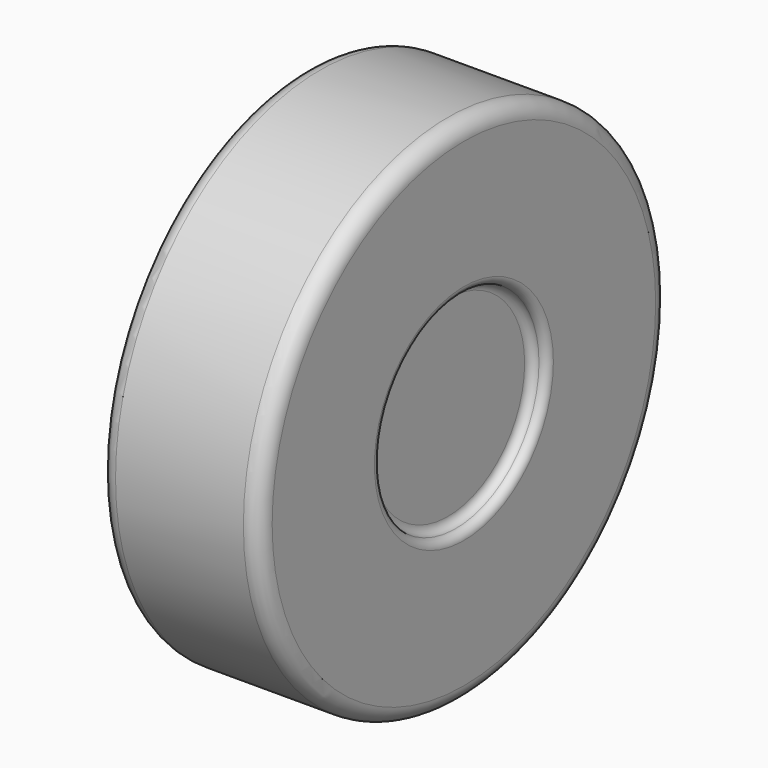
from build123d import *

# Parameters (mm, degrees)
F0_R     = 80
F1_DEPTH = 50
F2_R     = 32.5
F3_DEPTH = 5
F4_R     = 32.5
F5_DEPTH = 25
F6_R     = 5
F7_DEPTH = 10
F8_R     = 5
F9_R     = 2.49999


# Not quite as in the source:
# - a fillet or chamfer is up to 0.001 mm smaller than in the source, because OpenCascade refuses the exact size


with BuildPart() as f1:
    # F0 (on Right) → F1 (new body)
    with BuildSketch(Plane.YZ):
        Circle(F0_R)
    extrude(amount=F1_DEPTH)

    # F2 (on face) → F3 (cut)
    with BuildSketch(Plane.YZ.offset(50)):
        Circle(F2_R)
    extrude(amount=-F3_DEPTH, mode=Mode.SUBTRACT)

    # F4 (on face) → F5 (cut)
    with BuildSketch(Plane(origin=(0, 0, 0), x_dir=(0, -1, 0), z_dir=(-1, 0, 0))):
        Circle(F4_R)
    extrude(amount=-F5_DEPTH, mode=Mode.SUBTRACT)

    # F6 (on face) → F7 (cut)
    with BuildSketch(Plane(origin=(25, 0, 0), x_dir=(0, -1, 0), z_dir=(-1, 0, 0))):
        Circle(F6_R)
    extrude(amount=-F7_DEPTH, mode=Mode.SUBTRACT)

    # F8
    f8_edges = [f1.edges().sort_by_distance(p)[0] for p in [
        (0, -80, 0),
        (50, -80, 0),
    ]]
    fillet(f8_edges, radius=F8_R)

    # F9 (radius 2.5 in the source; OpenCascade refuses exactly that, so slightly less here)
    f9_edges = [f1.edges().sort_by_distance(p)[0] for p in [
        (50, -32.5, 0),
        (45, -32.5, 0),
        (0, 32.5, 0),
        (25, 32.5, 0),
    ]]
    fillet(f9_edges, radius=F9_R)


solid = f1.part
